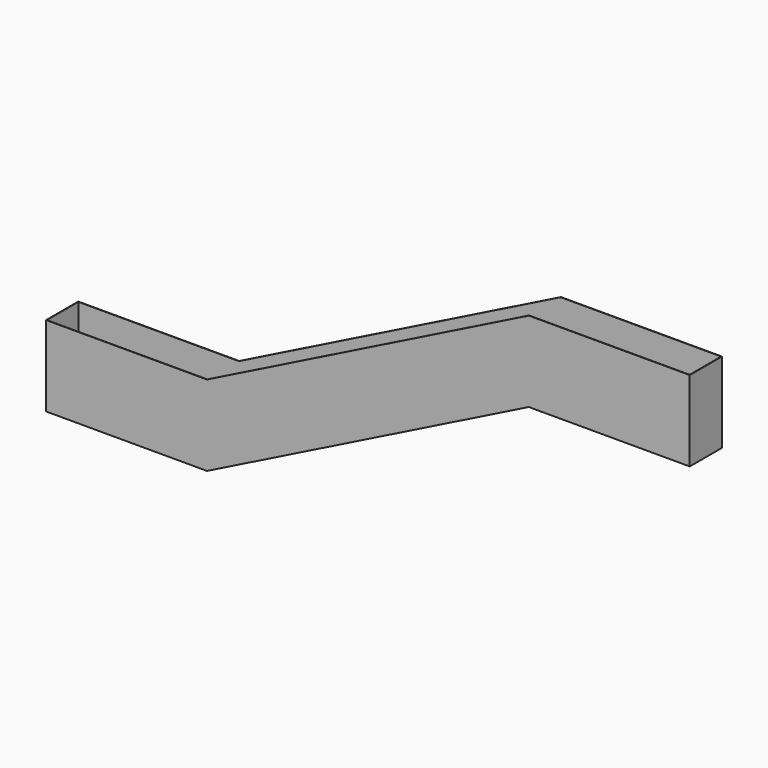
from build123d import *

# Parameters (mm, degrees)
F1_DEPTH = 100
F2_T     = -1
F5_D     = 20


# Not quite as in the source:
# - the program builds the solid bodies; features that only make, move or delete a surface that nothing else refers to are left out


with BuildPart() as f1:
    # F0 (on Front) → F1 (new body)
    with BuildSketch(Plane.XZ):
        Polygon((0, 200), (0, 0), (400, 0), (1200, 400), (1600, 400), (1600, 600), (1200, 600), (400, 200), align=None)
    extrude(amount=F1_DEPTH)

    # F2
    f2_openings = [f1.faces().sort_by_distance(p)[0] for p in [
        (200, -50, 200),
        (800, -50, 400),
        (1400, -50, 600),
    ]]
    offset(amount=F2_T, openings=f2_openings, kind=Kind.INTERSECTION)

    # F5 (through all)
    with Locations(Plane.XY.offset(401)):
        with Locations((1587, -13), (1587, -87)):
            Hole(F5_D / 2)


solid = f1.part
